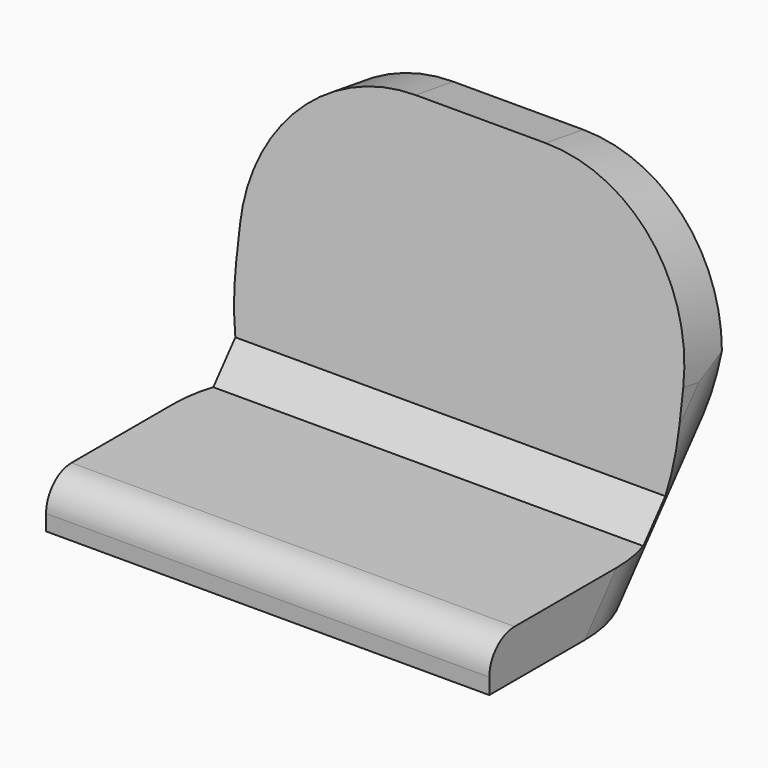
from build123d import *

# Parameters (mm, degrees)
F0_W        = 28
F0_H        = 3
F3_R        = 9.8982756057
F4_R        = 2
F5_T1_DEPTH = 29.9393718709
F5_T3_DEPTH = 39.6309025582
F5_T5_DEPTH = 35.0165294795


# Not quite as in the source:
# - a fillet or chamfer that OpenCascade refuses, or shapes differently, is made with other operations: its cross-section is extruded or revolved along the edge and cut away or added


with BuildPart() as f2:
    # F2: sweep along a path in F1
    with BuildLine(Plane.YZ) as f2_path:
        Line((0, 0), (13.3813479915, 0))
        Line((13.3813479915, 0), (15.8422850072, 2.9223633464))
        Line((15.8422850072, 2.9223633464), (18.3032229543, 18.9184583724))
    # F0 (on Front) → F2 (sweep)
    with BuildSketch(Plane.XZ):
        Rectangle(F0_W, F0_H)
    sweep(path=f2_path.line, transition=Transition.RIGHT)

    # F3
    f3_edges = [f2.edges().sort_by_distance(p)[0] for p in [
        (14, 18.303223, 18.918458),
        (-14, 18.303223, 18.918458),
    ]]
    fillet(f3_edges, radius=F3_R)

    # F4
    f4_edges = [f2.edges().sort_by_distance(p)[0] for p in [
        (0, 0, 1.5),
    ]]
    fillet(f4_edges, radius=F4_R)

    # F5: fillet of radius 5 on 4 edges, made by hand

    # F5_s2 → F5_t1 (cut)
    with BuildSketch(Plane(origin=(0, -2.9491433719, -3.5021085214), x_dir=(1, 0, 0), z_dir=(0, 0.6441356632, 0.7649112677))):
        with BuildLine():
            ThreePointArc((-9, 11.7355438551), (-12.5355339059, 10.271077761), (-14, 6.7355438551))
            Line((-14, 6.7355438551), (-14, 11.7355438551))
            Line((-14, 11.7355438551), (-9, 11.7355438551))
        make_face()
        with BuildLine():
            ThreePointArc((14, 6.7355438551), (12.5355339059, 10.271077761), (9, 11.7355438551))
            Line((9, 11.7355438551), (14, 11.7355438551))
            Line((14, 11.7355438551), (14, 6.7355438551))
        make_face()
    extrude(amount=F5_T1_DEPTH, mode=Mode.SUBTRACT)

    # F5_s4 → F5_t3 (cut)
    with BuildSketch(Plane.YZ.offset(-19.8154512791)):
        with BuildLine():
            ThreePointArc((11.7530216334, -1.5), (13.8621219652, -1.0333978195), (15.5775779716, 0.279321684))
            Line((15.5775779716, 0.279321684), (14.079202145, -1.5))
            Line((14.079202145, -1.5), (11.7530216334, -1.5))
        make_face()
    extrude(amount=F5_T3_DEPTH, mode=Mode.SUBTRACT)

    # F5_s6 → F5_t5 (cut)
    with BuildSketch(Plane.YZ.offset(-17.5082647397)):
        with BuildLine():
            ThreePointArc((16.356908347, 1.2047767074), (17.0849215873, 2.3580628903), (17.4742104853, 3.6651690265))
            Line((17.4742104853, 3.6651690265), (17.2608277209, 2.2781811991))
            Line((17.2608277209, 2.2781811991), (16.356908347, 1.2047767074))
        make_face()
    extrude(amount=F5_T5_DEPTH, mode=Mode.SUBTRACT)


solid = f2.part
